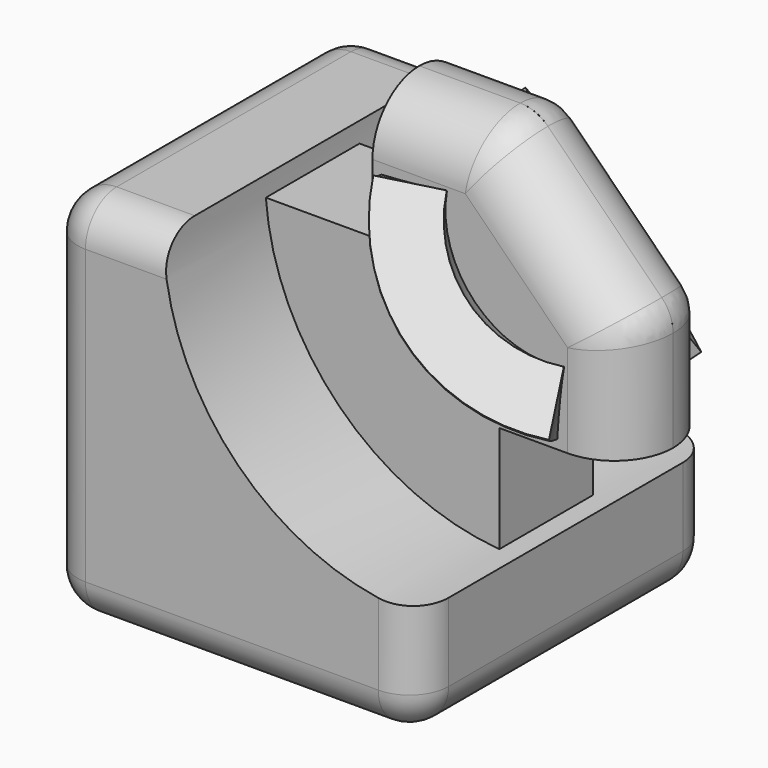
from build123d import *

# Parameters (mm, degrees)
F0_W           = 19
F0_H           = 19
F1_DEPTH       = 9.5
F3_DEPTH       = 19.001
F5_DEPTH       = 3
F6_R           = 2
F8_DEPTH       = 12.501
F9_R           = 2
F10_R          = 2.99999
F11_R          = 2
F13_ANGLE_BACK = 50
F13_ANGLE      = 100


# Not quite as in the source:
# - a fillet or chamfer is up to 0.001 mm smaller than in the source, because OpenCascade refuses the exact size


with BuildPart() as f1:
    # F0 (on Front) → F1 (new body, symmetric)
    with BuildSketch(Plane.XZ):
        with Locations((9.5, 9.5)):
            Rectangle(F0_W, F0_H)
    extrude(amount=F1_DEPTH, both=True)

    # F2 (on face) → F3 (cut, through all)
    with BuildSketch(Plane.XZ.offset(9.5)):
        with BuildLine():
            ThreePointArc((6, 19), (9.8076118446, 9.8076118446), (19, 6))
            Line((19, 6), (19, 19))
            Line((19, 19), (6, 19))
        make_face()
    extrude(amount=-F3_DEPTH, mode=Mode.SUBTRACT)

    # F4 (on Front) → F5 (join, symmetric)
    with BuildSketch(Plane.XZ):
        Polygon((0, 18), (0, 0), (18, 0), (18, 11.5), (24.5, 11.5), (24.5, 24.5), (11.5, 24.5), (11.5, 18), align=None)
    extrude(amount=F5_DEPTH, both=True)

    # F6
    f6_edges = [f1.edges().sort_by_distance(p)[0] for p in [
        (0, 0, 0),
    ]]
    fillet(f6_edges, radius=F6_R)

    # F7 (on face) → F8 (cut, through all)
    with BuildSketch(Plane.XZ.offset(3)):
        Polygon((17.5, 24.5), (24.5, 17.5), (24.5, 24.5), align=None)
    extrude(amount=-F8_DEPTH, mode=Mode.SUBTRACT)

    # F9
    f9_edges = [f1.edges().sort_by_distance(p)[0] for p in [
        (0, -9.5, 10.5),
        (0, 9.5, 10.5),
        (0, 0, 19),
        (3, 9.5, 19),
        (3, -9.5, 19),
        (19, 9.5, 3),
        (19, 0, 0),
        (19, -9.5, 3),
    ]]
    fillet(f9_edges, radius=F9_R)

    # F10 (radius 3 in the source; OpenCascade refuses exactly that, so slightly less here)
    f10_edges = [f1.edges().sort_by_distance(p)[0] for p in [
        (14.5, -3, 24.5),
        (21, -3, 21),
        (24.5, -3, 14.5),
        (14.5, 3, 24.5),
        (21, 3, 21),
        (24.5, 3, 14.5),
    ]]
    fillet(f10_edges, radius=F10_R)

    # F11
    f11_edges = [f1.edges().sort_by_distance(p)[0] for p in [
        (17.118519, 2.162797, 23.579023),
        (23.579023, 2.162797, 17.118519),
    ]]
    fillet(f11_edges, radius=F11_R)

    # F12 (on Front) → F13 (revolve)
    with BuildSketch(Plane.XZ, mode=Mode.PRIVATE) as f13_sk:
        with BuildLine():
            Line((14.434, 20.434), (11.434, 20.434))
            ThreePointArc((11.434, 20.434), (14.0700389693, 14.0700389693), (20.434, 11.434))
            Line((20.434, 11.434), (20.434, 14.434))
            ThreePointArc((20.434, 14.434), (16.1913593129, 16.1913593129), (14.434, 20.434))
        make_face()
    revolve(f13_sk.sketch.rotate(Axis((20.434, 0, 20.434), (0.7071067812, 0, -0.7071067812)), -F13_ANGLE_BACK), axis=Axis((20.434, 0, 20.434), (0.7071067812, 0, -0.7071067812)), revolution_arc=F13_ANGLE)


solid = f1.part
